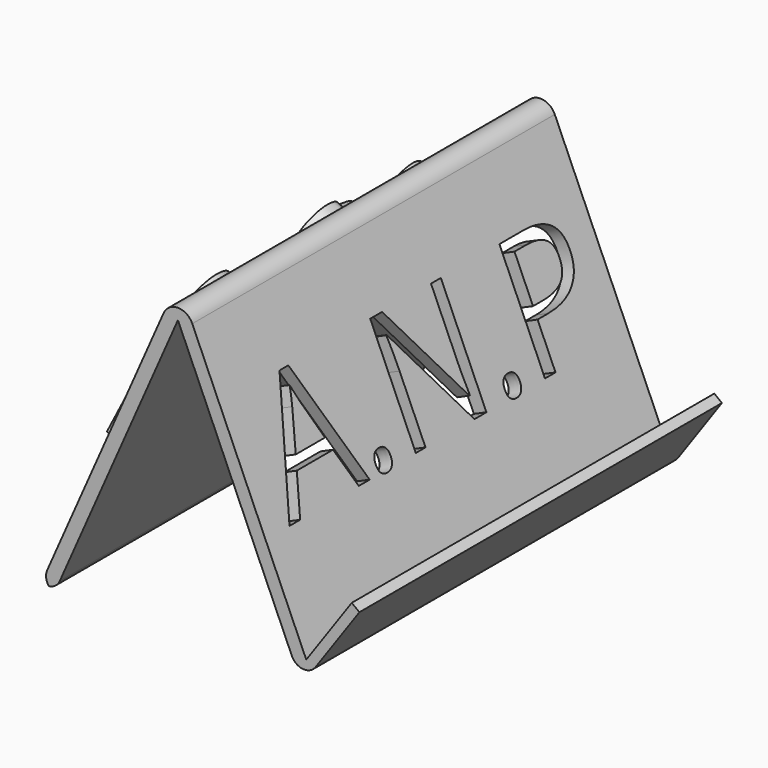
from build123d import *

# Parameters (mm, degrees)
F1_DEPTH     = 168.91
F2_R         = 5.8359239273
F3_T1_DEPTH  = 213.9549152378
F3_T3_DEPTH  = 194.31
F4_TEXT_SIZE = 59.010166054
F5_DEPTH     = 25.4
F7_DEPTH     = 7.62


# Not quite as in the source:
# - a fillet or chamfer that OpenCascade refuses, or shapes differently, is made with other operations: its cross-section is extruded or revolved along the edge and cut away or added
# - Text() gives the source's letters only with a copy of the font that has no kerning and outlines rounded to 1/6400 em; it was checked with that copy


with BuildPart() as f1:
    # F0 (on Front) → F1 (new body)
    with BuildSketch(Plane.XZ):
        Polygon((-50.7641643829, -43.0054690899), (-46.0817106068, -45.068923384), (0, 59.5011077821), (46.0817106068, -45.068923384), (67.6316011631, -14.3537702391), (64.7993334978, -12.1776337779), (47.8345812708, -36.3575692332), (0, 72.190129809), align=None)
    extrude(amount=F1_DEPTH)

    # F2
    f2_edges = [f1.edges().sort_by_distance(p)[0] for p in [
        (0, -84.455, 72.19013),
    ]]
    fillet(f2_edges, radius=F2_R)

    # F3: fillet of radius 5.08 on 3 edges, made by hand

    # F3_s2 → F3_t1 (cut)
    with BuildSketch(Plane.XZ.offset(-22.5224576189)):
        with BuildLine():
            ThreePointArc((51.2559619088, -37.6940404008), (46.598519036, -39.8318194496), (42.4487631154, -36.8249275036))
            Line((42.4487631154, -36.8249275036), (46.0817106068, -45.068923384))
            Line((46.0817106068, -45.068923384), (51.2559619088, -37.6940404008))
        make_face()
    extrude(amount=F3_T1_DEPTH, mode=Mode.SUBTRACT)

    # F3_s4 → F3_t3 (cut)
    with BuildSketch(Plane.XZ.offset(-12.7)):
        with BuildLine():
            ThreePointArc((-50.7303483999, -43.0203710491), (-46.8432580059, -43.1073618104), (-44.033158272, -40.4202855908))
            Line((-44.033158272, -40.4202855908), (-46.0817106068, -45.068923384))
            Line((-46.0817106068, -45.068923384), (-50.7303483999, -43.0203710491))
        make_face()
        with BuildLine():
            ThreePointArc((-48.7156120481, -38.3568312968), (-48.8026028093, -42.2439216908), (-46.1155265898, -45.0540214247))
            Line((-46.1155265898, -45.0540214247), (-50.7641643829, -43.0054690899))
            Line((-50.7641643829, -43.0054690899), (-48.7156120481, -38.3568312968))
        make_face()
    extrude(amount=F3_T3_DEPTH, mode=Mode.SUBTRACT)

    # F4 (on face) → F5 (cut)
    with BuildSketch(Plane(origin=(26.6393221797, 0, 11.7393628151), x_dir=(0, 1, 0), z_dir=(0.9150861797, 0, 0.4032583336))):
        with Locations((-157.7513664961, -14.9463806301)):
            Text('A.N.P', F4_TEXT_SIZE, font='Open Sans', text_align=(TextAlign.LEFT, TextAlign.BOTTOM))
    extrude(amount=-F5_DEPTH, mode=Mode.SUBTRACT)


with BuildPart() as f7:
    # F6 (on face) → F7 (new body)
    with BuildSketch(Plane(origin=(-26.6393221797, 0, 11.7393628151), x_dir=(0, -1, 0), z_dir=(-0.9150861797, 0, 0.4032583336))):
        with BuildLine():
            add(Edge.make_bspline(
                [(71.8945860863, 16.6349448264), (72.4843129144, 18.0995712866), (73.7008926935, 21.1210294438), (76.0081367462, 26.2403108427), (75.42542807, 30.4248401284), (75.1228928566, 32.5973965228)],
                knots=[0, 0, 0, 0, 0.3114538868, 0.6425152845, 1, 1, 1, 1], degree=3))
            add(Edge.make_bspline(
                [(71.8945860863, 16.6349448264), (70.9131923013, 16.3954106538), (68.4965102782, 15.8055577958), (61.2784563796, 18.1359298651), (56.3169656562, 23.9001308393), (50.5482536321, 31.7099497532), (45.2931460662, 38.3350602486), (40.112346845, 41.2999305009), (35.0410566934, 40.9586627359), (30.5518917076, 36.9105979984), (26.4970018265, 31.638912231), (23.459016238, 24.9331194107), (20.0025892531, 14.7517648495), (17.538765929, 4.6475737468), (16.4638677834, -5.2390649982), (15.8745404333, -10.6595475227)],
                knots=[0, 0, 0, 0, 0.0505734886, 0.1245372069, 0.2017384965, 0.2890013525, 0.3702317839, 0.4361270773, 0.495715523, 0.5627776796, 0.6342117394, 0.7097622026, 0.8001424503, 0.8904254132, 1, 1, 1, 1], degree=3))
            add(Edge.make_bspline(
                [(15.8745404333, -10.6595475227), (16.1938379433, -9.8163104223), (16.7721698158, -8.2889859809), (17.2863289918, -7.2114598531), (17.5166204572, -6.7288368009)],
                knots=[0, 0, 0, 0, 0.5521008356, 1, 1, 1, 1], degree=3))
            add(Edge.make_bspline(
                [(17.5166204572, -6.7288368009), (17.4011675213, -7.2786051141), (17.1599673002, -8.4271617769), (19.1241377682, -9.4524583137), (21.2073227142, -9.0484889807), (22.8421066552, -6.7363942267), (23.438105023, -5.8343432845), (23.6939731985, -5.4470836185)],
                knots=[0, 0, 0, 0, 0.1797513413, 0.3755301928, 0.5805534743, 0.8199273302, 1, 1, 1, 1], degree=3))
            add(Edge.make_bspline(
                [(23.6939731985, -5.4470836185), (23.5374566609, -6.2890349102), (23.2417500366, -7.8797331078), (25.3532954298, -9.1189281956), (26.6712445009, -8.2266870523), (27.3691061884, -7.754240185)],
                knots=[0, 0, 0, 0, 0.3460040867, 0.6537053656, 1, 1, 1, 1], degree=3))
            add(Edge.make_bspline(
                [(27.3691061884, -7.754240185), (27.5303701231, -8.1961480845), (27.8649066103, -9.112870826), (29.3621217373, -10.2659776036), (31.5667487525, -9.2750931236), (31.9575884049, -8.2363032558), (32.1389622986, -7.754240185)],
                knots=[0, 0, 0, 0, 0.2304709133, 0.4781039845, 0.7578078073, 1, 1, 1, 1], degree=3))
            add(Edge.make_bspline(
                [(32.1389622986, -7.754240185), (32.0024470922, -8.5021014051), (31.7395350324, -9.9423932158), (33.6758672853, -11.060425732), (35.0736486515, -10.5749288064), (35.8140952885, -10.3177465498)],
                knots=[0, 0, 0, 0, 0.3368331917, 0.6487006875, 1, 1, 1, 1], degree=3))
            add(Edge.make_bspline(
                [(35.8140952885, -10.3177465498), (35.7500019355, -10.8238620163), (35.6085928625, -11.9405038463), (36.7759022613, -14.3333675917), (38.722748664, -14.3922440459), (40.4590577459, -13.6144167324), (40.867902805, -12.8157878152), (41.0531125963, -12.4540030956)],
                knots=[0, 0, 0, 0, 0.19329834, 0.4264738511, 0.626541934, 0.8308207745, 1, 1, 1, 1], degree=3))
            add(Edge.make_bspline(
                [(41.0531125963, -12.4540030956), (41.0207927492, -13.0158925595), (40.9505464595, -14.2371437006), (41.5301343996, -17.104971865), (44.2710432637, -17.1377335376), (45.495066411, -15.8605291565), (46.1434461176, -15.183978714)],
                knots=[0, 0, 0, 0, 0.2242509481, 0.4874032062, 0.7284713451, 1, 1, 1, 1], degree=3))
            add(Edge.make_bspline(
                [(46.1434461176, -15.183978714), (46.0689802959, -15.7404157976), (45.8958575118, -17.0340554143), (47.3653440154, -20.3157798067), (49.5057015139, -20.4052449225), (51.2175985507, -19.0478500723), (51.706262931, -17.8729702978), (51.9456155598, -17.2975026071)],
                knots=[0, 0, 0, 0, 0.186615551, 0.4338554656, 0.6163800265, 0.8120991568, 1, 1, 1, 1], degree=3))
            add(Edge.make_bspline(
                [(51.9456155598, -17.2975026071), (52.0199071645, -18.3582848839), (52.1626133246, -20.3959332313), (54.828668268, -22.3478900075), (56.3712836896, -20.8357611927), (56.9020605971, -19.9220461389), (57.1617074311, -19.4750726223)],
                knots=[0, 0, 0, 0, 0.2945761824, 0.5658490761, 0.787620917, 1, 1, 1, 1], degree=3))
            add(Edge.make_bspline(
                [(57.1617074311, -19.4750726223), (57.3946993058, -20.6897170083), (57.7907077257, -22.754207045), (59.6456689413, -23.0995161794), (61.9781740587, -22.7736366312), (63.0129908749, -19.4711136571), (63.3154998791, -18.5969704339), (63.4327381849, -18.2581935078)],
                knots=[0, 0, 0, 0, 0.240718297, 0.4091407588, 0.6047174992, 0.8468070368, 1, 1, 1, 1], degree=3))
            add(Edge.make_bspline(
                [(63.4327381849, -18.2581935078), (63.6946399017, -18.9964076989), (64.2232998646, -20.4865250286), (66.3196040584, -22.4873673489), (69.101291853, -21.1372059168), (70.3498124798, -18.2509748749), (70.5752080506, -14.4035810553), (70.5195129334, -11.8682209518), (70.4916878311, -10.6015631615)],
                knots=[0, 0, 0, 0, 0.1489809665, 0.3007245359, 0.4545128264, 0.6225176955, 0.8114110492, 1, 1, 1, 1], degree=3))
            Line((70.4916878311, -10.6015631615), (71.5248957276, -8.0372430384))
            ThreePointArc((71.5248957276, -8.0372430384), (72.2442346037, -10.6546048584), (73.3576565981, -13.1301498041))
            ThreePointArc((73.3576565981, -13.1301498041), (72.0463054368, -21.8220107052), (67.2833621502, -29.2100049555))
            add(Edge.make_bspline(
                [(67.2833621502, -29.2100049555), (67.1901868014, -29.3428971554), (66.9946151297, -29.6218330544), (67.0670681525, -30.0047092429), (67.1050027013, -30.2051734179)],
                knots=[0, 0, 0, 0, 0.4764255886, 1, 1, 1, 1], degree=3))
            Line((67.1050027013, -30.2051734179), (59.5783106983, -33.8716953993))
            Line((59.5783106983, -33.8716953993), (53.3995181322, -31.9634787738))
            add(Edge.make_bspline(
                [(53.3995181322, -31.9634787738), (53.1039743193, -31.6361120894), (52.4188225653, -30.8771861763), (50.067467231, -30.0375756914), (47.7343815738, -30.3225774904), (46.5390516484, -31.4268348667), (45.9216329262, -32.9415806826), (47.0723307126, -34.3051345725), (49.1291597167, -35.3292978237), (50.7748583099, -35.5523071272), (51.7622913603, -35.0751479297), (52.2552840412, -34.8369181156)],
                knots=[0, 0, 0, 0, 0.0987781939, 0.2289949911, 0.3547637285, 0.4586717802, 0.5575769579, 0.6625960364, 0.7893956808, 0.8948522253, 1, 1, 1, 1], degree=3))
            Line((52.2552840412, -34.8369181156), (55.7464919984, -35.2857597172))
            Line((55.7464919984, -35.2857597172), (53.2821081579, -36.1273400486))
            add(Edge.make_bspline(
                [(53.2821081579, -36.1273400486), (52.89903083, -36.1088741238), (52.0558186955, -36.0682277825), (50.2933370003, -36.4144915502), (49.0419915544, -37.3764272497), (48.049595351, -38.4216372402), (47.8590640068, -39.6870548982), (49.1580130822, -41.3554549868), (51.8237548885, -41.0328364235), (53.3473449722, -40.4050188676), (54.3173720428, -39.3367288768), (54.8350661993, -38.766592741)],
                knots=[0, 0, 0, 0, 0.0948896706, 0.2088667636, 0.3175400673, 0.4187657564, 0.5105963098, 0.6262817502, 0.7621712287, 0.8730730627, 1, 1, 1, 1], degree=3))
            Line((54.8350661993, -38.766592741), (58.1116937101, -36.2480953336))
            Line((58.1116937101, -36.2480953336), (57.0138096809, -39.6759919822))
            add(Edge.make_bspline(
                [(57.0138096809, -39.6759919822), (56.5859238783, -39.9402960277), (55.6644728734, -40.5094741281), (54.4078105463, -42.3872977023), (54.7282067023, -44.1762980262), (56.3892351217, -46.213563181), (59.9724512008, -44.1828529867), (60.3986425244, -41.4226750499), (60.0491430546, -40.7172685642), (59.9153675139, -40.4472649097)],
                knots=[0, 0, 0, 0, 0.1266084626, 0.2726510072, 0.4051560896, 0.5505032753, 0.7376630059, 0.8995870487, 1, 1, 1, 1], degree=3))
            Line((59.9153675139, -40.4472649097), (61.1700937152, -35.6482118368))
            Line((61.1700937152, -35.6482118368), (68.9337253571, -32.9058989882))
            ThreePointArc((68.9337253571, -32.9058989882), (77.321810209, -31.9483709895), (82.6014205813, -25.3603104502))
            ThreePointArc((82.6014205813, -25.3603104502), (84.5289826393, -25.6676114431), (86.4565446973, -25.3603104502))
            ThreePointArc((86.4565446973, -25.3603104502), (92.0102743793, -31.9071640877), (100.5474627018, -32.8135974705))
            Line((100.5474627018, -32.8135974705), (108.5474640131, -36.091979593))
            Line((108.5474640131, -36.091979593), (109.5474585891, -40.6618416309))
            add(Edge.make_bspline(
                [(109.5474585891, -40.6618416309), (109.3854902495, -40.9765420575), (109.0291938012, -41.6688171317), (109.4440464873, -43.2791096636), (110.8365026343, -44.8774106989), (112.8498869538, -45.8661082094), (114.5782138357, -44.6200477652), (115.1925729594, -42.8353483175), (114.4182049456, -40.9242280965), (113.1262383751, -40.0045623125), (112.4391183257, -39.5154468715)],
                knots=[0, 0, 0, 0, 0.0958466272, 0.2108425198, 0.3468877256, 0.4787099462, 0.6047737508, 0.7279057287, 0.8552892673, 1, 1, 1, 1], degree=3))
            Line((112.4391183257, -39.5154468715), (111.8173114624, -36.673859879))
            Line((111.8173114624, -36.673859879), (111.8424832821, -36.5199930966))
            Line((111.8424832821, -36.5199930966), (114.5589724183, -38.5402664542))
            add(Edge.make_bspline(
                [(114.5589724183, -38.5402664542), (114.7568508556, -38.96471676), (115.1856168858, -39.8844221867), (117.0286018589, -40.7479917584), (118.9990264557, -41.0694566638), (121.0745211795, -40.3797600664), (121.6197525558, -39.0658297673), (120.8965053681, -37.2824150771), (118.6758958901, -36.3907643022), (116.8692453352, -36.3673886831), (115.9172207117, -36.3550707698)],
                knots=[0, 0, 0, 0, 0.1080442564, 0.2341119503, 0.3642851138, 0.4931873258, 0.593406183, 0.7114854772, 0.8479656571, 1, 1, 1, 1], degree=3))
            Line((115.9172207117, -36.3550707698), (113.1630018353, -35.0376926363))
            Line((113.1630018353, -35.0376926363), (117.0786619186, -34.4960093498))
            add(Edge.make_bspline(
                [(115.9456521273, -32.0197306573), (116.5027662716, -31.5517150641), (117.6348283304, -30.6007022393), (119.9851667695, -29.7075675137), (122.3095221988, -30.9657759381), (123.6139375425, -31.8735082977), (122.7155675953, -34.5840223246), (120.7744569356, -35.3640595964), (118.0424553604, -35.2075026017), (117.3521380084, -34.697895339), (117.0786619186, -34.4960093498)],
                knots=[0, 0, 0, 0, 0.1299977524, 0.2641568603, 0.4029616807, 0.5051780331, 0.6394554265, 0.7651522275, 0.9069627175, 1, 1, 1, 1], degree=3))
            Line((115.9456521273, -32.0197306573), (109.9973917007, -33.7221734226))
            Line((109.9973917007, -33.7221734226), (103.0020043254, -29.9325976521))
            ThreePointArc((103.0020043254, -29.9325976521), (97.8022442842, -22.2892260674), (96.4565500617, -13.143312186))
            ThreePointArc((96.4565500617, -13.143312186), (97.6857254932, -10.6418473279), (98.0480536819, -7.878350094))
            Line((98.0480536819, -7.878350094), (99.0954339504, -10.196885094))
            add(Edge.make_bspline(
                [(99.0954339504, -10.196885094), (99.0715753213, -10.9944216666), (99.0168818672, -12.8226922577), (99.5240404295, -16.9331835267), (100.6303793783, -21.2958730358), (103.1058954381, -22.8267697018), (105.46067035, -21.5265633224), (105.9899373304, -19.763750514), (106.2689423561, -18.8344772905)],
                knots=[0, 0, 0, 0, 0.1521299938, 0.348742369, 0.5502287494, 0.698108269, 0.8408566692, 1, 1, 1, 1], degree=3))
            add(Edge.make_bspline(
                [(106.2689423561, -18.8344772905), (106.5902397586, -19.8391535153), (107.2065933196, -21.7664512902), (109.7082160852, -23.9859126774), (111.9495802, -21.8553578772), (112.3297378986, -20.501648542), (112.5125512481, -19.8506657034)],
                knots=[0, 0, 0, 0, 0.2763741502, 0.5301760623, 0.7740672147, 1, 1, 1, 1], degree=3))
            add(Edge.make_bspline(
                [(112.5125512481, -19.8506657034), (112.9993897609, -20.3382019331), (113.9144180023, -21.2545415555), (115.7096211304, -21.8230921585), (117.2680929274, -19.8378645605), (117.7265419164, -18.4016741747), (117.9591044784, -17.6731217653)],
                knots=[0, 0, 0, 0, 0.249530052, 0.4689995526, 0.7306334458, 1, 1, 1, 1], degree=3))
            add(Edge.make_bspline(
                [(117.9591044784, -17.6731217653), (118.4048440337, -18.589851008), (119.2027639878, -20.2308912673), (121.2348596808, -19.9509849476), (122.8036366845, -18.9511555432), (123.22260246, -16.6942837791), (123.4720796347, -15.3504079208)],
                knots=[0, 0, 0, 0, 0.2666498054, 0.4773307596, 0.6887716062, 1, 1, 1, 1], degree=3))
            add(Edge.make_bspline(
                [(123.4720796347, -15.3504079208), (123.9524702165, -15.8500038799), (124.893774097, -16.8289398389), (126.9259949855, -17.0750278714), (128.520208416, -16.028677787), (128.7916577818, -13.6810296652), (128.8132540808, -12.952554084), (128.8219243288, -12.6600936055)],
                knots=[0, 0, 0, 0, 0.2154450098, 0.4221548702, 0.6205494363, 0.8476623015, 1, 1, 1, 1], degree=3))
            add(Edge.make_bspline(
                [(128.8219243288, -12.6600936055), (129.3225588685, -13.187355708), (130.2453849054, -14.1592646713), (131.8138254204, -14.4082144916), (133.5358703174, -13.4879918187), (133.8745429313, -11.5285906488), (133.9593663563, -10.4747036473), (133.9999139309, -9.9709210917)],
                knots=[0, 0, 0, 0, 0.2172642022, 0.400485877, 0.6007709145, 0.8091591901, 1, 1, 1, 1], degree=3))
            add(Edge.make_bspline(
                [(133.9999139309, -9.9709210917), (134.5819530587, -10.4269843031), (135.6978686165, -11.3013723099), (137.3256272498, -10.034470271), (137.5697456895, -8.9817956034), (137.691155076, -8.4582604468)],
                knots=[0, 0, 0, 0, 0.3540087986, 0.6787240016, 1, 1, 1, 1], degree=3))
            add(Edge.make_bspline(
                [(137.691155076, -8.4582604468), (138.2863610076, -9.0566579571), (139.3860709294, -10.1622646797), (141.7088150956, -10.3838332443), (142.1585614012, -8.5318706581), (142.4077302217, -7.5058448128)],
                knots=[0, 0, 0, 0, 0.3447603909, 0.6369836093, 1, 1, 1, 1], degree=3))
            add(Edge.make_bspline(
                [(142.4077302217, -7.5058448128), (143.0720488559, -8.0488849399), (144.3098985634, -9.0607518783), (145.6605798082, -7.5016042355), (146.0435519846, -6.6319165355), (146.2302803993, -6.2078768387)],
                knots=[0, 0, 0, 0, 0.3724653246, 0.6940285421, 1, 1, 1, 1], degree=3))
            add(Edge.make_bspline(
                [(146.2302803993, -6.2078768387), (146.8160862831, -6.9723851736), (147.9578099142, -8.46239621), (150.6402276011, -10.9313511248), (151.9578878344, -8.6847136991), (152.6492983103, -7.5058448128)],
                knots=[0, 0, 0, 0, 0.3337004754, 0.6503753701, 1, 1, 1, 1], degree=3))
            add(Edge.make_bspline(
                [(152.6492983103, -7.5058448128), (153.2209416231, -8.7134322772), (153.7925849358, -9.9210197416), (154.3642282486, -11.128607206)],
                knots=[0, 0, 0, 0, 4.0081656716, 4.0081656716, 4.0081656716, 4.0081656716], degree=3))
            add(Edge.make_bspline(
                [(154.3642282486, -11.128607206), (153.8777124807, -7.5191637619), (153.1064616061, -1.7972805334), (152.6396331505, 1.0754194675), (148.3159166814, 29.2941262884), (135.6874504533, 43.4815242067), (121.6213340814, 41.6700334887), (117.9228200129, 27.8977273162), (108.5740339225, 18.3617513796), (101.4696989604, 17.1376816671), (98.1172770262, 16.5600627661)],
                knots=[0, 0, 0, 0, 0.1082329215, 0.1715766289, 0.3582081963, 0.5119018152, 0.6284345134, 0.7578586125, 0.8857373557, 1, 1, 1, 1], degree=3))
            add(Edge.make_bspline(
                [(98.1172770262, 16.5600627661), (97.6308405779, 19.0635880277), (96.5604383955, 24.5725890769), (91.7267714613, 35.3878641695), (88.9950024468, 42.1306593179), (81.7628143964, 46.3198212793), (74.7706305525, 44.5669859613), (74.1679101351, 42.6944226089), (73.9411041141, 41.9897697866)],
                knots=[0, 0, 0, 0, 0.1807321689, 0.3977006837, 0.5681220511, 0.7440820543, 0.9036970886, 1, 1, 1, 1], degree=3))
            add(Edge.make_bspline(
                [(73.9411041141, 41.9897697866), (72.1863438819, 41.6422089342), (68.8981924284, 40.9909332207), (65.2509049215, 39.3895182077), (62.7461090557, 36.1682272669), (63.7606973492, 33.7938017591), (64.2719194293, 32.5973965228)],
                knots=[0, 0, 0, 0, 0.2830032766, 0.5303047211, 0.7633339562, 1, 1, 1, 1], degree=3))
            add(Edge.make_bspline(
                [(64.2719194293, 32.5973965228), (64.6648701739, 33.1736009505), (65.558852573, 34.4844945517), (69.1714906422, 33.8694660305), (72.9283493163, 33.0664644534), (75.1228928566, 32.5973965228)],
                knots=[0, 0, 0, 0, 0.2459372106, 0.5595193307, 1, 1, 1, 1], degree=3))
        make_face()
    extrude(amount=F7_DEPTH)


solid = Compound([f1.part, f7.part])
